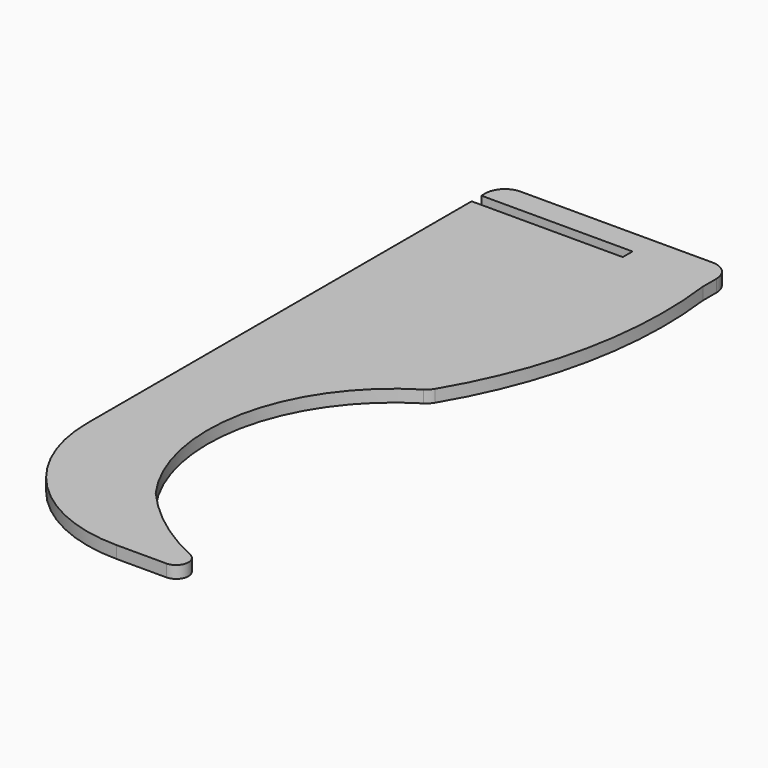
from build123d import *

# Parameters (mm, degrees)
F1_DEPTH = 3.175
F2_R     = 5.08


# Not quite as in the source:
# - a length typed as a fraction of an inch, garbled in the dataset ("3 / 203.2 mm" for 3/8 in), is restored


with BuildPart() as f1:
    # F0 (on Top) → F1 (new body)
    with BuildSketch(Plane.XY):
        with BuildLine():
            Line((0, 6.35), (0, 0))
            Line((0, 0), (39.228014, 0))
            Line((39.228014, 0), (39.228014, -3.175))
            Line((39.228014, -3.175), (0, -3.175))
            Line((0, -3.175), (0, -30.5298216847))
            Line((0, -30.5298216847), (0, -127.8741553825))
            ThreePointArc((0, -127.8741553825), (11.1624656807, -154.8181574015), (38.1091467085, -165.9741542846))
            Line((38.1091467085, -165.9741542846), (51.0104592901, -165.9710570523))
            ThreePointArc((51.0104592901, -165.9710570523), (54.1114045686, -163.4743163552), (52.3355938941, -159.9111615484))
            ThreePointArc((52.3355938941, -159.9111615484), (40.2763953072, -152.7327194477), (30, -143.175))
            ThreePointArc((30, -143.175), (22.0311793243, -104.8602527123), (45, -73.175))
            ThreePointArc((45, -73.175), (58.4492609505, -39.4498416322), (60, -3.175))
            Line((60, -3.175), (60, 0))
            Line((60, 0), (60, 6.35))
            Line((60, 6.35), (39.228014, 6.35))
            Line((39.228014, 6.35), (0, 6.35))
        make_face()
    extrude(amount=F1_DEPTH)

    # F2
    f2_edges = [f1.edges().sort_by_distance(p)[0] for p in [
        (60, 6.35, 1.5875),
        (0, 6.35, 1.5875),
        (45, -73.175, 1.5875),
    ]]
    fillet(f2_edges, radius=F2_R)


solid = f1.part
